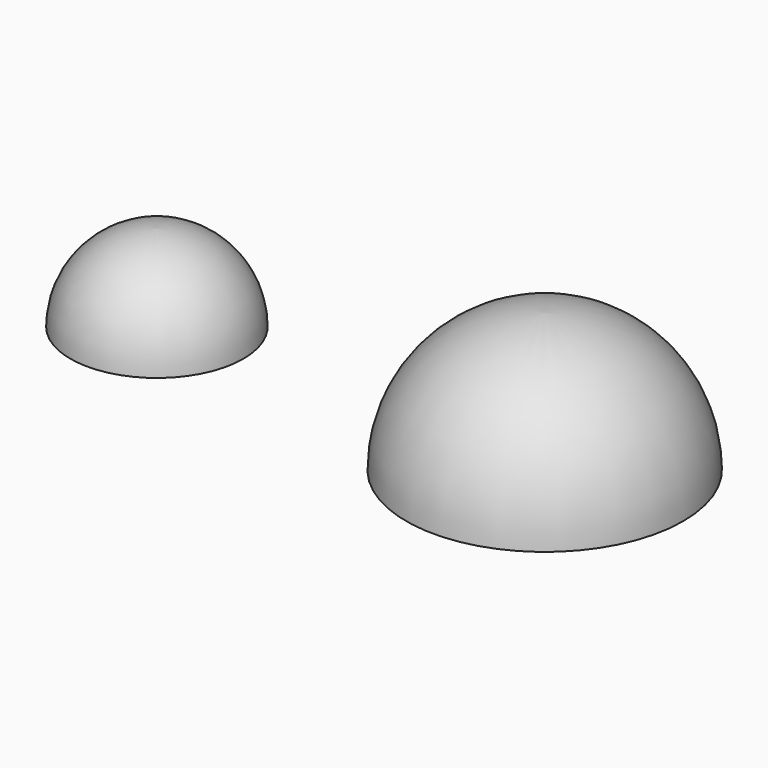
from build123d import *

# Parameters (mm, degrees)
F0_R     = 2.5
F1_DEPTH = 2.5
F0_R_2   = 4
F2_DEPTH = 4
F3_R     = 2.49999
F4_R     = 3.99999


# Not quite as in the source:
# - a fillet or chamfer is up to 0.001 mm smaller than in the source, because OpenCascade refuses the exact size


with BuildPart() as f1:
    # F0 (on Top) → F1 (new body)
    with BuildSketch(Plane.XY):
        Circle(F0_R)
    extrude(amount=F1_DEPTH)

    # F3 (radius 2.5 in the source; OpenCascade refuses exactly that, so slightly less here)
    f3_edges = [f1.edges().sort_by_distance(p)[0] for p in [
        (-2.5, 0, 2.5),
    ]]
    fillet(f3_edges, radius=F3_R)


with BuildPart() as f2:
    # F0 (on Top) → F2 (new body)
    with BuildSketch(Plane.XY):
        with Locations((11.2059488893, 0)):
            Circle(F0_R_2)
    extrude(amount=F2_DEPTH)

    # F4 (radius 4 in the source; OpenCascade refuses exactly that, so slightly less here)
    f4_edges = [f2.edges().sort_by_distance(p)[0] for p in [
        (7.205949, 0, 4),
    ]]
    fillet(f4_edges, radius=F4_R)


solid = Compound([f1.part, f2.part])
